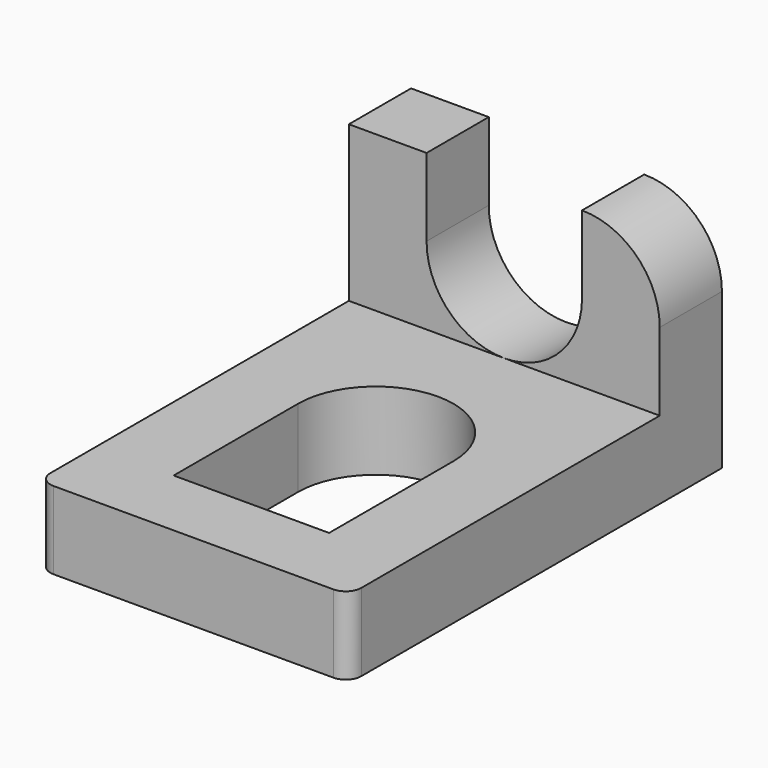
from build123d import *

# Parameters (mm, degrees)
F0_W     = 4
F0_H     = 5
F1_DEPTH = 1
F2_R     = 0.2
F3_R     = 0.2
F5_DEPTH = 25
F7_DEPTH = 1
F8_R     = 0.99999


# Not quite as in the source:
# - a fillet or chamfer is up to 0.001 mm smaller than in the source, because OpenCascade refuses the exact size


with BuildPart() as f1:
    # F0 (on Top) → F1 (new body)
    with BuildSketch(Plane.XY):
        with Locations((2, 2.5)):
            Rectangle(F0_W, F0_H)
    extrude(amount=F1_DEPTH)

    # F2
    f2_edges = [f1.edges().sort_by_distance(p)[0] for p in [
        (4, 0, 0.5),
    ]]
    fillet(f2_edges, radius=F2_R)

    # F3
    f3_edges = [f1.edges().sort_by_distance(p)[0] for p in [
        (0, 0, 0.5),
    ]]
    fillet(f3_edges, radius=F3_R)

    # F4 (on face) → F5 (cut)
    with BuildSketch(Plane.XY.offset(1)):
        with BuildLine():
            Line((1, 2.9323451086), (1, 0.9323451086))
            Line((1, 0.9323451086), (3, 0.9323451086))
            Line((3, 0.9323451086), (3, 2.9323451086))
            ThreePointArc((3, 2.9323451086), (2, 3.9323451086), (1, 2.9323451086))
        make_face()
    extrude(amount=-F5_DEPTH, mode=Mode.SUBTRACT)

    # F6 (on face) → F7 (join)
    with BuildSketch(Plane(origin=(0, 5, 0), x_dir=(-1, 0, 0), z_dir=(0, 1, 0))):
        with BuildLine():
            Line((-4, 3), (-4, 1))
            Line((-4, 1), (-4, 0))
            Line((-4, 0), (0, 0))
            Line((0, 0), (0, 1))
            Line((0, 1), (0, 3))
            Line((0, 3), (-1, 3))
            Line((-1, 3), (-1, 2))
            ThreePointArc((-1, 2), (-2, 1), (-3, 2))
            Line((-3, 2), (-3, 3))
            Line((-3, 3), (-4, 3))
        make_face()
    extrude(amount=F7_DEPTH)

    # F8 (radius 1 in the source; OpenCascade refuses exactly that, so slightly less here)
    f8_edges = [f1.edges().sort_by_distance(p)[0] for p in [
        (4, 5.5, 3),
    ]]
    fillet(f8_edges, radius=F8_R)


solid = f1.part
